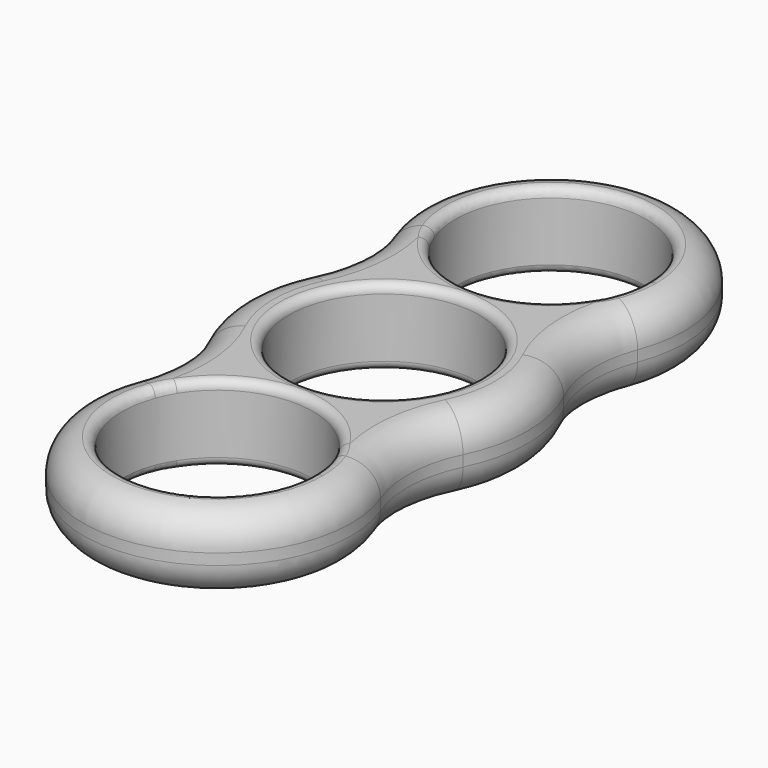
from build123d import *

# Parameters (mm, degrees)
F0_R     = 11.049
F1_DEPTH = 8.89
F2_R     = 3.81
F3_R     = 1.01599


# Not quite as in the source:
# - a fillet or chamfer is up to 0.001 mm smaller than in the source, because OpenCascade refuses the exact size


with BuildPart() as f1:
    # F0 (on Top) → F1 (new body)
    with BuildSketch(Plane.XY):
        with BuildLine():
            ThreePointArc((-14.9783819929, -7.2840320572), (-13.5550662693, -12.8953460907), (-14.4774998386, -18.6103954468))
            ThreePointArc((-14.4774998386, -18.6103954468), (0, -39.624), (14.4774998386, -18.6103954468))
            ThreePointArc((14.4774998386, -18.6103954468), (13.5550662693, -12.8953460907), (14.9783819929, -7.2840320572))
            ThreePointArc((14.9783819929, -7.2840320572), (16.655601164, 0), (14.9783819929, 7.2840320572))
            ThreePointArc((14.9783819929, 7.2840320572), (13.5550662693, 12.8953460907), (14.4774998386, 18.6103954468))
            ThreePointArc((14.4774998386, 18.6103954468), (0, 39.624), (-14.4774998386, 18.6103954468))
            ThreePointArc((-14.4774998386, 18.6103954468), (-13.5550662693, 12.8953460907), (-14.9783819929, 7.2840320572))
            ThreePointArc((-14.9783819929, 7.2840320572), (-16.655601164, 0), (-14.9783819929, -7.2840320572))
        make_face()
        with Locations((0, -24.13)):
            Circle(F0_R, mode=Mode.SUBTRACT)
        Circle(F0_R, mode=Mode.SUBTRACT)
        with Locations((0, 24.13)):
            Circle(F0_R, mode=Mode.SUBTRACT)
    extrude(amount=F1_DEPTH)

    # F2
    f2_edges = [f1.edges().sort_by_distance(p)[0] for p in [
        (13.555066, -12.895346, 0),
        (0, -39.624, 8.89),
    ]]
    fillet(f2_edges, radius=F2_R)

    # F3 (radius 1.016 in the source; OpenCascade refuses exactly that, so slightly less here)
    f3_edges = [f1.edges().sort_by_distance(p)[0] for p in [
        (-11.049, -24.13, 8.89),
        (-11.049, 0, 8.89),
        (-11.049, 24.13, 8.89),
        (-11.049, 24.13, 0),
        (-11.049, 0, 0),
        (-11.049, -24.13, 0),
    ]]
    fillet(f3_edges, radius=F3_R)


solid = f1.part
